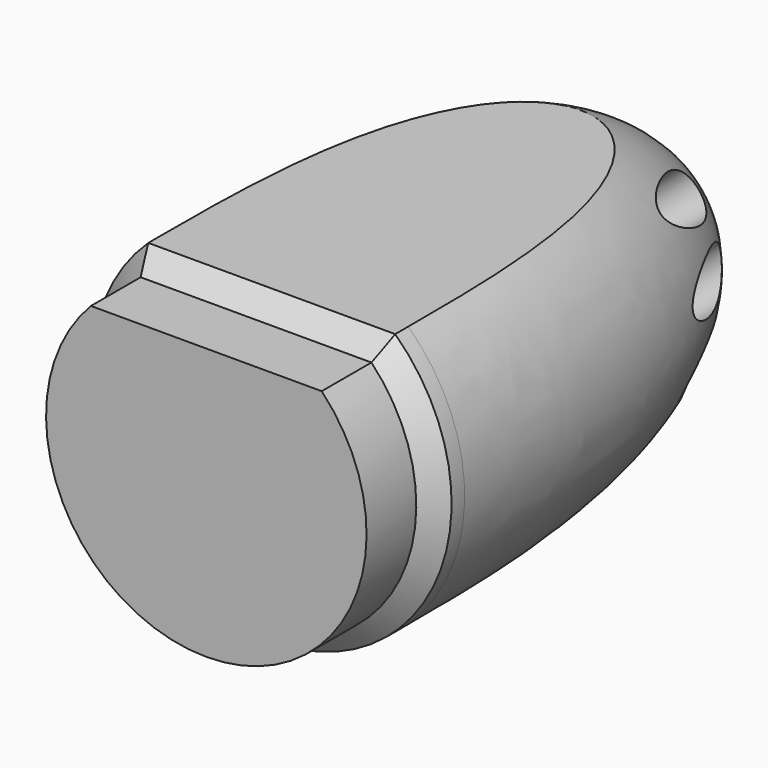
from build123d import *

# Parameters (mm, degrees)
F2_W     = 60
F2_H     = 6
F3_DEPTH = 22
F5_DEPTH = 10
F6_SIZE  = 2.39999
F7_R     = 3
F7_R_2   = 5.5
F8_DEPTH = 40


# Not quite as in the source:
# - a fillet or chamfer is up to 0.001 mm smaller than in the source, because OpenCascade refuses the exact size


with BuildPart() as f1:
    # F0 (on Right) → F1 (revolve)
    with BuildSketch(Plane.YZ):
        with BuildLine():
            Line((0, 22), (0, 0))
            Line((0, 0), (70, 0))
            Line((70, 0), (70, 5))
            add(Edge.make_bspline(
                [(12, 22), (32, 22), (60, 22), (70, 5)],
                knots=[0, 0, 0, 0, 60.440052945, 60.440052945, 60.440052945, 60.440052945], degree=3))
            Line((12, 22), (0, 22))
        make_face()
    revolve(axis=Axis((0, 35, 0), (0, 1, 0)))

    # F2 (on Right) → F3 (cut, symmetric)
    with BuildSketch(Plane.YZ):
        with Locations((30, 19)):
            Rectangle(F2_W, F2_H)
    extrude(amount=F3_DEPTH, both=True, mode=Mode.SUBTRACT)

    # F4 (on face) → F5 (cut)
    with BuildSketch(Plane.XZ):
        with BuildLine():
            Line((15.0996688705, 16), (-15.0996688705, 16))
            ThreePointArc((-15.0996688705, 16), (0, -22), (15.0996688705, 16))
        make_face()
        with BuildLine():
            ThreePointArc((14.1138230115, 13.6), (0, -19.6), (-14.1138230115, 13.6))
            Line((-14.1138230115, 13.6), (14.1138230115, 13.6))
        make_face(mode=Mode.SUBTRACT)
    extrude(amount=-F5_DEPTH, mode=Mode.SUBTRACT)

    # F6 (size 2.4 in the source; OpenCascade refuses exactly that, so slightly less here)
    f6_edges = [f1.edges().sort_by_distance(p)[0] for p in [
        (0, 10, -19.6),
        (0, 10, 13.6),
    ]]
    chamfer(f6_edges, length=F6_SIZE)

    # F7 (on face) → F8 (cut)
    with BuildSketch(Plane(origin=(0, 70, 0), x_dir=(-1, 0, 0), z_dir=(0, 1, 0))):
        with Locations((11.4906666468, 9.6418141453)):
            Circle(F7_R)
        with Locations((14.8716729206, 1.9578928833)):
            Circle(F7_R)
        with Locations((13.5946168055, -6.3392739261)):
            Circle(F7_R)
        with Locations((8.0594941252, -12.6508716872)):
            Circle(F7_R)
        with Locations((0, -15)):
            Circle(F7_R)
        with Locations((-8.0594941252, -12.6508716872)):
            Circle(F7_R)
        with Locations((-13.5946168055, -6.3392739261)):
            Circle(F7_R)
        with Locations((-14.8716729206, 1.9578928833)):
            Circle(F7_R)
        with Locations((-11.4906666468, 9.6418141453)):
            Circle(F7_R)
        Circle(F7_R_2)
    extrude(amount=-F8_DEPTH, mode=Mode.SUBTRACT)


solid = f1.part
